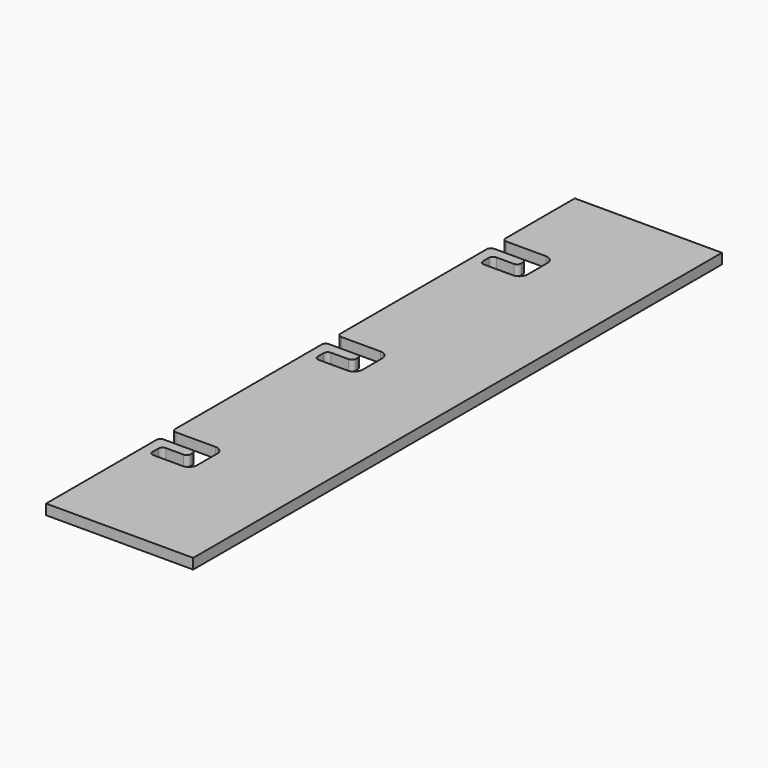
from build123d import *

# Parameters (mm, degrees)
F1_DEPTH = 3.175


# Not quite as in the source:
# - a length typed as a fraction of an inch, garbled in the dataset ("3 / 203.2 mm" for 3/8 in), is restored


with BuildPart() as f1:
    # F0 (on Top) → F1 (new body)
    with BuildSketch(Plane.XY):
        with BuildLine():
            Line((0, 0), (0, 203.2))
            Line((0, 203.2), (-45.24375, 203.2))
            Line((-45.24375, 203.2), (-45.24375, 176.68875))
            ThreePointArc((-45.24375, 176.68875), (-44.8717756121, 175.7907243879), (-43.97375, 175.41875))
            Line((-43.97375, 175.41875), (-31.90875, 175.41875))
            ThreePointArc((-31.90875, 175.41875), (-30.1126987758, 174.6748012242), (-29.36875, 172.87875))
            Line((-29.36875, 172.87875), (-29.36875, 165.25875))
            ThreePointArc((-29.36875, 165.25875), (-30.1126987758, 163.4626987758), (-31.90875, 162.71875))
            Line((-31.90875, 162.71875), (-40.79875, 162.71875))
            ThreePointArc((-40.79875, 162.71875), (-41.6967756121, 163.0907243879), (-42.06875, 163.98875))
            Line((-42.06875, 163.98875), (-42.06875, 166.21125))
            ThreePointArc((-42.06875, 166.21125), (-41.6967756121, 167.1092756121), (-40.79875, 167.48125))
            Line((-40.79875, 167.48125), (-35.40125, 167.48125))
            ThreePointArc((-35.40125, 167.48125), (-34.5032243879, 167.8532243879), (-34.13125, 168.75125))
            Line((-34.13125, 168.75125), (-34.13125, 169.38625))
            ThreePointArc((-34.13125, 169.38625), (-34.5032243879, 170.2842756121), (-35.40125, 170.65625))
            Line((-35.40125, 170.65625), (-43.97375, 170.65625))
            ThreePointArc((-43.97375, 170.65625), (-44.8717756121, 170.2842756121), (-45.24375, 169.38625))
            Line((-45.24375, 169.38625), (-45.24375, 113.18875))
            ThreePointArc((-45.24375, 113.18875), (-44.8717756121, 112.2907243879), (-43.97375, 111.91875))
            Line((-43.97375, 111.91875), (-31.90875, 111.91875))
            ThreePointArc((-31.90875, 111.91875), (-30.1126987758, 111.1748012242), (-29.36875, 109.37875))
            Line((-29.36875, 109.37875), (-29.36875, 101.75875))
            ThreePointArc((-29.36875, 101.75875), (-30.1126987758, 99.9626987758), (-31.90875, 99.21875))
            Line((-31.90875, 99.21875), (-40.79875, 99.21875))
            ThreePointArc((-40.79875, 99.21875), (-41.6967756121, 99.5907243879), (-42.06875, 100.48875))
            Line((-42.06875, 100.48875), (-42.06875, 102.71125))
            ThreePointArc((-42.06875, 102.71125), (-41.6967756121, 103.6092756121), (-40.79875, 103.98125))
            Line((-40.79875, 103.98125), (-35.40125, 103.98125))
            ThreePointArc((-35.40125, 103.98125), (-34.5032243879, 104.3532243879), (-34.13125, 105.25125))
            Line((-34.13125, 105.25125), (-34.13125, 105.88625))
            ThreePointArc((-34.13125, 105.88625), (-34.5032243879, 106.7842756121), (-35.40125, 107.15625))
            Line((-35.40125, 107.15625), (-43.97375, 107.15625))
            ThreePointArc((-43.97375, 107.15625), (-44.8717756121, 106.7842756121), (-45.24375, 105.88625))
            Line((-45.24375, 105.88625), (-45.24375, 49.68875))
            ThreePointArc((-45.24375, 49.68875), (-44.8717756121, 48.7907243879), (-43.97375, 48.41875))
            Line((-43.97375, 48.41875), (-31.90875, 48.41875))
            ThreePointArc((-31.90875, 48.41875), (-30.1126987758, 47.6748012242), (-29.36875, 45.87875))
            Line((-29.36875, 45.87875), (-29.36875, 38.25875))
            ThreePointArc((-29.36875, 38.25875), (-30.1126987758, 36.4626987758), (-31.90875, 35.71875))
            Line((-31.90875, 35.71875), (-40.79875, 35.71875))
            ThreePointArc((-40.79875, 35.71875), (-41.6967756121, 36.0907243879), (-42.06875, 36.98875))
            Line((-42.06875, 36.98875), (-42.06875, 39.21125))
            ThreePointArc((-42.06875, 39.21125), (-41.6967756121, 40.1092756121), (-40.79875, 40.48125))
            Line((-40.79875, 40.48125), (-35.40125, 40.48125))
            ThreePointArc((-35.40125, 40.48125), (-34.5032243879, 40.8532243879), (-34.13125, 41.75125))
            Line((-34.13125, 41.75125), (-34.13125, 42.38625))
            ThreePointArc((-34.13125, 42.38625), (-34.5032243879, 43.2842756121), (-35.40125, 43.65625))
            Line((-35.40125, 43.65625), (-43.97375, 43.65625))
            ThreePointArc((-43.97375, 43.65625), (-44.8717756121, 43.2842756121), (-45.24375, 42.38625))
            Line((-45.24375, 42.38625), (-45.24375, 0))
            Line((-45.24375, 0), (0, 0))
        make_face()
    extrude(amount=F1_DEPTH)


solid = f1.part
